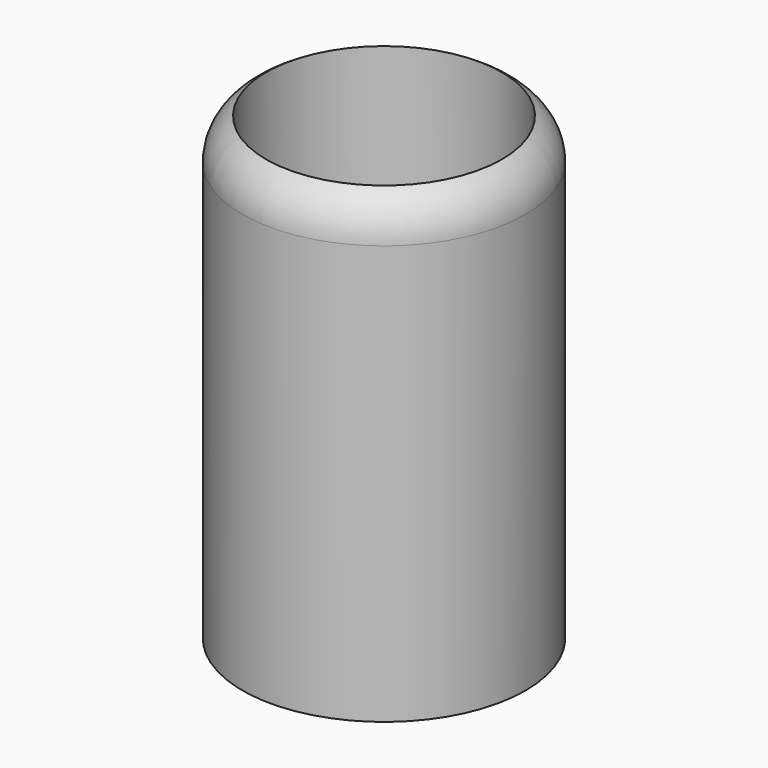
from build123d import *

# Parameters (mm, degrees)
F0_R     = 38.1
F0_R_2   = 31.75
F1_DEPTH = 123.825
F2_DEPTH = 114.3


# Not quite as in the source:
# - a fillet or chamfer that OpenCascade refuses, or shapes differently, is made with other operations: its cross-section is extruded or revolved along the edge and cut away or added


with BuildPart() as f1:
    # F0 (on Top) → F1 (new body)
    with BuildSketch(Plane.XY):
        Circle(F0_R)
        Circle(F0_R_2, mode=Mode.SUBTRACT)
        Circle(F0_R_2)
    extrude(amount=-F1_DEPTH)

    # F0 (on Top) → F2 (cut)
    with BuildSketch(Plane.XY):
        Circle(F0_R_2)
    extrude(amount=-F2_DEPTH, mode=Mode.SUBTRACT)

    # F3: fillet of radius 12.7 on 1 edges, made by hand

    # F3_s1 → F3_t2 (revolve, cut)
    with BuildSketch(Plane.XZ):
        with BuildLine():
            ThreePointArc((38.1, -10.9985226281), (36.3985226281, -4.6485226281), (31.75, 0))
            Line((31.75, 0), (38.1, 0))
            Line((38.1, 0), (38.1, -10.9985226281))
        make_face()
    revolve(axis=Axis((0, 0, 0), (0, 0, 1)), mode=Mode.SUBTRACT)


solid = f1.part
